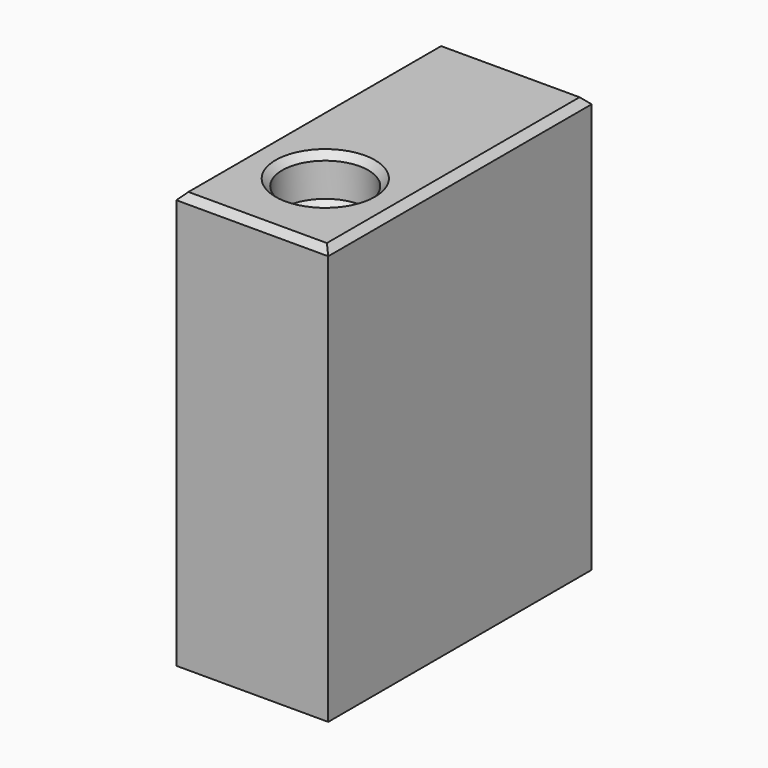
from build123d import *

# Parameters (mm, degrees)
F0_W         = 11.3
F0_H         = 24.5
F0_W_2       = 8.1
F0_H_2       = 21.3
F1_DEPTH     = 1
F2_DEPTH     = 6
F3_R         = 3.2
F4_DEPTH     = 24
F5_DEPTH     = 28.9
F8_R         = 0.5
F9_SIZE      = 0.5
F10_R        = 3.2
F10_R_2      = 2.25
F11_DEPTH    = 12
F12_S5_R     = 3.2
F12_T6_DEPTH = 6
F13_SIZE     = 1


# Not quite as in the source:
# - a fillet or chamfer that OpenCascade refuses, or shapes differently, is made with other operations: its cross-section is extruded or revolved along the edge and cut away or added


with BuildPart() as f1:
    # F0 (on Top) → F1 (new body)
    with BuildSketch(Plane.XY):
        Rectangle(F0_W, F0_H)
        Rectangle(F0_W_2, F0_H_2, mode=Mode.SUBTRACT)
        Rectangle(F0_W_2, F0_H_2)
    extrude(amount=F1_DEPTH)

    # F0 (on Top) → F2 (join)
    with BuildSketch(Plane.XY):
        Rectangle(F0_W, F0_H)
        Rectangle(F0_W_2, F0_H_2, mode=Mode.SUBTRACT)
    extrude(amount=-F2_DEPTH)

    # F3 (on face) → F4 (join)
    with BuildSketch(Plane.XY.offset(1)):
        with BuildLine():
            ThreePointArc((-5.65, -5.4622520893), (1e-08, -11.1122520693), (5.65, -5.4622520693))
            ThreePointArc((5.65, -5.4622520693), (-1e-08, 0.1877479307), (-5.65, -5.4622520893))
        make_face()
        with Locations((0, -5.4622520693)):
            Circle(F3_R, mode=Mode.SUBTRACT)
        with BuildLine():
            Line((5.65, -12.25), (5.65, -5.4622520693))
            ThreePointArc((5.65, -5.4622520693), (1e-08, -11.1122520693), (-5.65, -5.4622520893))
            Line((-5.65, -5.4622520893), (-5.65, -12.25))
            Line((-5.65, -12.25), (5.65, -12.25))
        make_face()
        with BuildLine():
            ThreePointArc((-5.65, -5.4622520893), (-1e-08, 0.1877479307), (5.65, -5.4622520693))
            Line((5.65, -5.4622520693), (5.65, 12.25))
            Line((5.65, 12.25), (-5.65, 12.25))
            Line((-5.65, 12.25), (-5.65, -5.4622520893))
        make_face()
    extrude(amount=F4_DEPTH)

    # F5 (cut): a face of the model
    f5_faces = [f1.faces().sort_by_distance(p)[0] for p in [
        (0, -5.4622520693, 1),
    ]]
    extrude(f5_faces, amount=-F5_DEPTH, mode=Mode.SUBTRACT)

    # F6 (on Right) → F7 (revolve)
    with BuildSketch(Plane.YZ):
        Polygon((-8.6622520693, 22), (-8.6622520693, 20), (-7.6622520693, 21), align=None)
    revolve(axis=Axis((0, -5.4622520693, 1), (0, 0, -1)))

    # F8
    f8_edges = [f1.edges().sort_by_distance(p)[0] for p in [
        (0, -3.262252, 21),
    ]]
    fillet(f8_edges, radius=F8_R)

    # F9
    f9_edges = [f1.edges().sort_by_distance(p)[0] for p in [
        (-5.65, 0, 25),
        (0, -12.25, 25),
        (5.65, 0, 25),
        (0, 12.25, 25),
        (-3.2, -5.462252, 25),
    ]]
    chamfer(f9_edges, length=F9_SIZE)

    # F10 (on face) → F11 (join)
    with BuildSketch(Plane.XY):
        with Locations((0, -5.4622520693)):
            Circle(F10_R)
        with Locations((0, -5.4622520693)):
            Circle(F10_R_2, mode=Mode.SUBTRACT)
    extrude(amount=F11_DEPTH)

    # F12: chamfer of 1 on 1 edges, made by hand


with BuildPart() as f12_tool2:
    # F12_s3 → F12_t4 (revolve)
    with BuildSketch(Plane.XZ.offset(5.4622520693)):
        Polygon((3.25, 12), (2.25, 11), (2.25, 12), align=None)
    revolve(axis=Axis((0, -5.4622520693, 12), (0, 0, 1)))

    # F12_s5 → F12_t6 (intersect, symmetric)
    with BuildSketch(Plane.XY.offset(11.5)):
        with Locations((0, -5.4622520693)):
            Circle(F12_S5_R)
    extrude(amount=F12_T6_DEPTH, both=True, mode=Mode.INTERSECT)


with BuildPart() as f1_1:
    add(f1.part)

    # F12_t1: cut F12_tool2
    add(f12_tool2.part, mode=Mode.SUBTRACT)

    # F13
    f13_edges = [f1_1.edges().sort_by_distance(p)[0] for p in [
        (-2.25, -5.462252, 0),
    ]]
    chamfer(f13_edges, length=F13_SIZE)


solid = f1_1.part
